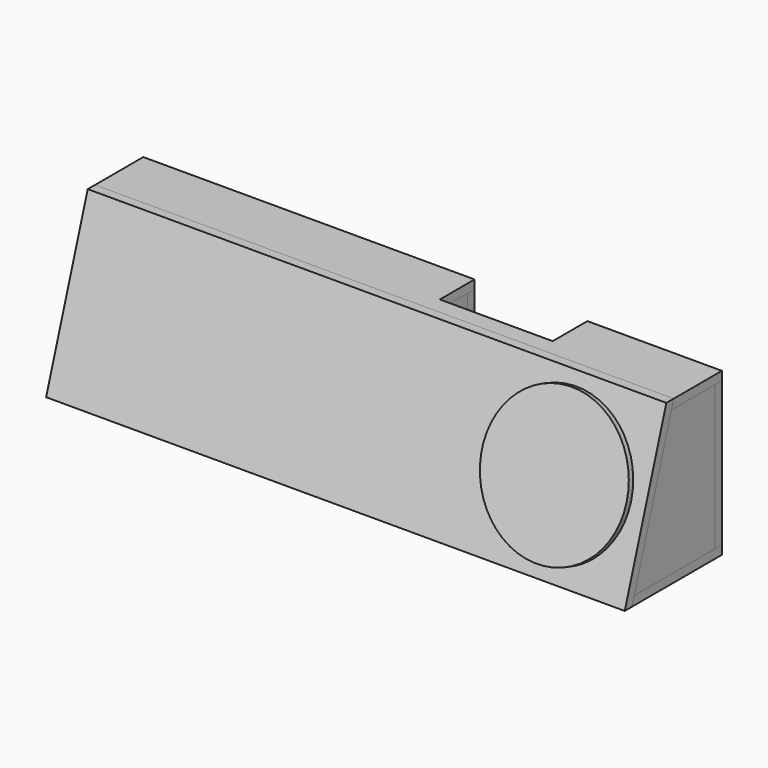
from build123d import *

# Parameters (mm, degrees)
F1_DEPTH  = 1270
F0_W      = 19.05
F0_H      = 317.5
F2_DEPTH  = 295.275
F3_W      = 19.05
F3_H      = 317.5
F4_DEPTH  = 727.075
F6_DEPTH  = 50.8
F7_W      = 285.75
F7_H      = 19.05
F8_DEPTH  = 127
F9_W      = 285.75
F9_H      = 95.25
F10_DEPTH = 139.7
F11_DEPTH = 1270
F12_DEPTH = 1270
F13_R     = 140.49375
F14_DEPTH = 25.4
F15_R     = 69.85
F16_DEPTH = 168.91
F17_R     = 158.75
F18_DEPTH = 12.7
F19_DEPTH = 19.05
F21_DEPTH = 19.05
F22_DEPTH = 660.4
F23_W     = 247.65
F23_H     = 127
F24_DEPTH = 19.05
F25_W     = 247.65
F25_H     = 107.95
F26_DEPTH = 31.75
F28_DEPTH = 19.05
F29_W     = 247.65
F29_H     = 76.2
F30_DEPTH = 120.65


with BuildPart() as f1:
    # F0 (on Right) → F1 (new body)
    with BuildSketch(Plane.YZ):
        Polygon((-20.3388575805, -22.6093402624), (-26.4620718662, -41.6593402624), (220.2280242562, -41.6593402624), (220.2280242562, -22.6093402624), (201.1780242562, -22.6093402624), align=None)
    extrude(amount=-F1_DEPTH)

    # F23 (on face) → F24 (cut)
    with BuildSketch(Plane(origin=(0, 0, -41.6593402624), x_dir=(1, 0, 0), z_dir=(0, 0, -1))):
        with Locations((-419.1, -156.7280242562)):
            Rectangle(F23_W, F23_H)
    extrude(amount=-F24_DEPTH, mode=Mode.SUBTRACT)


with BuildPart() as f2:
    # F0 (on Right) → F2 (new body)
    with BuildSketch(Plane.YZ):
        with Locations((210.7030242562, 136.1406597376)):
            Rectangle(F0_W, F0_H)
    extrude(amount=-F2_DEPTH)


with BuildPart() as f4:
    # F3 (on face) → F4 (new body)
    with BuildSketch(Plane(origin=(-1270, 0, 0), x_dir=(0, -1, 0), z_dir=(-1, 0, 0))):
        with Locations((-210.7030242562, 136.1406597376)):
            Rectangle(F3_W, F3_H)
    extrude(amount=-F4_DEPTH)


with BuildPart() as f6:
    # F5 (on face) → F6 (new body)
    with BuildSketch(Plane.XY.offset(-22.6093402624)):
        Polygon((-276.225, 201.1780242562), (-542.925, 201.1780242562), (-561.975, 201.1780242562), (-561.975, 74.1780242562), (-276.225, 74.1780242562), align=None)
    extrude(amount=F6_DEPTH)

    # F7 (on face) → F8 (join)
    with BuildSketch(Plane.XY.offset(28.1906597376)):
        with Locations((-419.1, 191.6530242562)):
            Rectangle(F7_W, F7_H)
    extrude(amount=F8_DEPTH)

    # F9 (on face) → F10 (join)
    with BuildSketch(Plane.XY.offset(155.1906597376)):
        with Locations((-419.1, 153.5530242562)):
            Rectangle(F9_W, F9_H)
    extrude(amount=F10_DEPTH)

    # F25 (on face) → F26 (cut)
    with BuildSketch(Plane(origin=(0, 0, -22.6093402624), x_dir=(1, 0, 0), z_dir=(0, 0, -1))):
        with Locations((-419.1, -147.2030242562)):
            Rectangle(F25_W, F25_H)
    extrude(amount=-F26_DEPTH, mode=Mode.SUBTRACT)

    # F29 (on face) → F30 (cut)
    with BuildSketch(Plane.XY.offset(294.8906597376)):
        with Locations((-419.1, 163.0780242562)):
            Rectangle(F29_W, F29_H)
    extrude(amount=-F30_DEPTH, mode=Mode.SUBTRACT)


with BuildPart() as f11:
    # F0 (on Right) → F11 (new body)
    with BuildSketch(Plane.YZ):
        Polygon((220.2280242562, 313.9406597376), (87.8379281338, 313.9406597376), (81.7147138481, 294.8906597376), (201.1780242562, 294.8906597376), (220.2280242562, 294.8906597376), align=None)
    extrude(amount=-F11_DEPTH)

    # F27 (on face) → F28 (cut)
    with BuildSketch(Plane.XY.offset(313.9406597376)):
        Polygon((-542.925, 201.1780242562), (-542.925, 124.9780242562), (-295.275, 124.9780242562), (-295.275, 201.1780242562), (-295.275, 220.2280242562), (-542.925, 220.2280242562), align=None)
    extrude(amount=-F28_DEPTH, mode=Mode.SUBTRACT)


with BuildPart() as f12:
    # F0 (on Right) → F12 (new body)
    with BuildSketch(Plane.YZ):
        Polygon((67.8280242562, 313.9406597376), (-46.4719757438, -41.6593402624), (-26.4620718662, -41.6593402624), (-20.3388575805, -22.6093402624), (81.7147138481, 294.8906597376), (87.8379281338, 313.9406597376), align=None)
    extrude(amount=-F12_DEPTH)

    # F13 (on face) → F14 (cut)
    with BuildSketch(Plane(origin=(0, -29.9836707942, 9.6376084696), x_dir=(1, 0, 0), z_dir=(0, -0.9520285613, 0.3060091804))):
        with Locations((-190.5, 132.8773698735)):
            Circle(F13_R)
    extrude(amount=-F14_DEPTH, mode=Mode.SUBTRACT)


with BuildPart() as f16:
    # F15 (on face) → F16 (new body)
    with BuildSketch(Plane(origin=(0, -29.9836707942, 9.6376084696), x_dir=(1, 0, 0), z_dir=(0, -0.9520285613, 0.3060091804))):
        with Locations((-190.5, 132.8773698735)):
            Circle(F15_R)
    extrude(amount=-F16_DEPTH)

    # F17 (on face) → F18 (join)
    with BuildSketch(Plane(origin=(0, -29.9836707942, 9.6376084696), x_dir=(1, 0, 0), z_dir=(0, -0.9520285613, 0.3060091804))):
        with Locations((-190.5, 132.8773698735)):
            Circle(F17_R)
    extrude(amount=F18_DEPTH)


with BuildPart() as f19:
    # F0 (on Right) → F19 (new body)
    with BuildSketch(Plane.YZ):
        Polygon((81.7147138481, 294.8906597376), (-20.3388575805, -22.6093402624), (201.1780242562, -22.6093402624), (201.1780242562, 294.8906597376), align=None)
    extrude(amount=-F19_DEPTH)


with BuildPart() as f21:
    # F20 (on face) → F21 (new body)
    with BuildSketch(Plane(origin=(-1270, 0, 0), x_dir=(0, -1, 0), z_dir=(-1, 0, 0))):
        Polygon((-201.1780242562, -22.6093402624), (-155.6353369512, -22.6093402624), (-33.510861462, 144.923118981), (-81.7147138481, 294.8906597376), (-201.1780242562, 294.8906597376), align=None)
    extrude(amount=-F21_DEPTH)


with BuildPart() as f22:
    # F20 (on face) → F22 (new body)
    with BuildSketch(Plane(origin=(-1270, 0, 0), x_dir=(0, -1, 0), z_dir=(-1, 0, 0))):
        Polygon((-155.6353369512, -22.6093402624), (-132.0611424195, -22.6093402624), (-26.2969415145, 122.4798124775), (-33.510861462, 144.923118981), align=None)
    extrude(amount=-F22_DEPTH)


solid = Compound([f1.part, f2.part, f4.part, f6.part, f11.part, f12.part, f16.part, f19.part, f21.part, f22.part])
